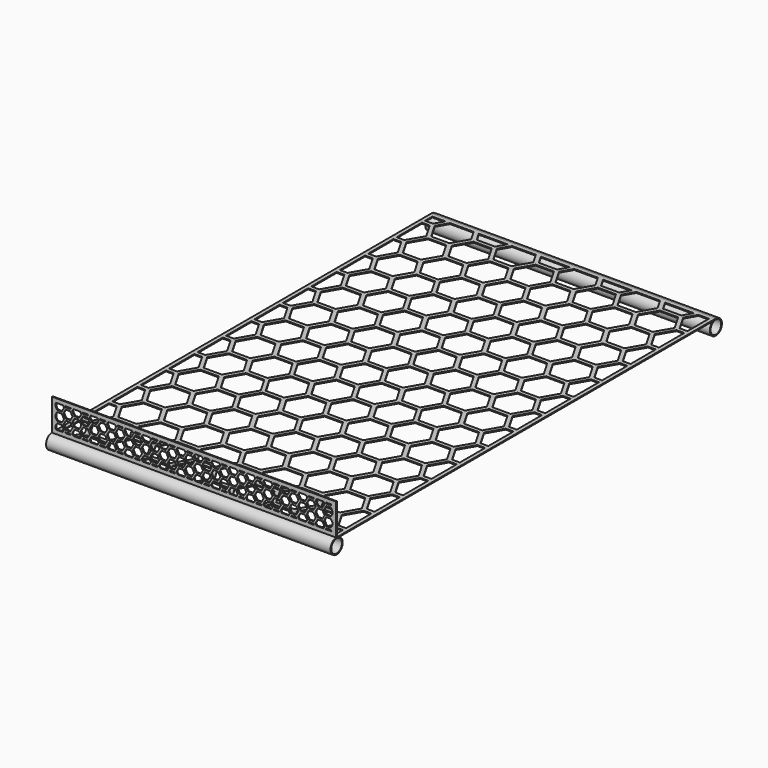
from build123d import *

# Parameters (mm, degrees)
F0_W     = 180
F0_H     = 300
F1_DEPTH = 0.3
F2_R     = 4.2
F2_R_2   = 4.8
F5_DEPTH = 0.6
F7_DEPTH = 490


# Not quite as in the source:
# - an extrude ends at something that could not be found from the text; its depth is read off the source's solid


with BuildPart() as f1:
    # F0 (on Top) → F1 (new body, symmetric)
    with BuildSketch(Plane.XY):
        Rectangle(F0_W, F0_H)
    extrude(amount=F1_DEPTH, both=True)

    # F3: sweep along a path in F3_path
    with BuildLine(Plane(origin=(-90, -150, 0.3), x_dir=(0, 1, 0), z_dir=(0, 0, 1))) as f3_path:
        Line((0, 0), (0, -180))
    # F2 (on Right) → F3 (sweep)
    with BuildSketch(Plane.YZ):
        with BuildLine():
            ThreePointArc((-150.3, 0.2906158268), (-153.286335345, -7.9985711369), (-145.2, -4.5))
            ThreePointArc((-145.2, -4.5), (-146.5014288631, -1.213664655), (-149.7, 0.2906158268))
            Line((-149.7, 0.2906158268), (-150.3, 0.2906158268))
        make_face()
        with Locations((-150, -4.5)):
            Circle(F2_R, mode=Mode.SUBTRACT)
        with BuildLine():
            Line((-150.3, 0.2906158268), (-149.7, 0.2906158268))
            ThreePointArc((-149.7, 0.2906158268), (-150, 0.3), (-150.3, 0.2906158268))
        make_face()
        with BuildLine():
            ThreePointArc((-150.3, 0.2906158268), (-150, 0.3), (-149.7, 0.2906158268))
            Line((-149.7, 0.2906158268), (-149.7, 20.2906158268))
            Line((-149.7, 20.2906158268), (-150.3, 20.2906158268))
            Line((-150.3, 20.2906158268), (-150.3, 0.2906158268))
        make_face()
        with Locations((150, -4.5)):
            Circle(F2_R_2)
        with Locations((150, -4.5)):
            Circle(F2_R, mode=Mode.SUBTRACT)
    sweep(path=f3_path.line)

    # F4 (on face) → F5 (cut, through all)
    with BuildSketch(Plane.XY.offset(0.3)):
        Polygon((-79.2319517736, 147.6762099923), (-87.5, 147.6762099923), (-87.5, 141.875), (-82.5812819243, 141.875), align=None)
        Polygon((-61.3932256344, 147.6762099923), (-76.3452004277, 147.6762099923), (-80.4162184149, 140.625), (-74.642715723, 130.625), (-63.0957103392, 130.625), (-57.3222076473, 140.625), align=None)
        Polygon((-39.9259517736, 147.6762099923), (-58.1716174588, 147.6762099923), (-54.8222873081, 141.875), (-43.2752819243, 141.875), align=None)
        Polygon((-22.0872256344, 147.6762099923), (-37.0392004277, 147.6762099923), (-41.1102184149, 140.625), (-35.336715723, 130.625), (-23.7897103392, 130.625), (-18.0162076473, 140.625), align=None)
        Polygon((-0.6199517736, 147.6762099923), (-18.8656174588, 147.6762099923), (-15.5162873081, 141.875), (-3.9692819243, 141.875), align=None)
        Polygon((17.2187743656, 147.6762099923), (2.2667995723, 147.6762099923), (-1.8042184149, 140.625), (3.969284277, 130.625), (15.5162896608, 130.625), (21.2897923527, 140.625), align=None)
        Polygon((38.6860482264, 147.6762099923), (20.4403825412, 147.6762099923), (23.7897126919, 141.875), (35.3367180757, 141.875), align=None)
        Polygon((56.5247743656, 147.6762099923), (41.5727995723, 147.6762099923), (37.5017815851, 140.625), (43.275284277, 130.625), (54.8222896608, 130.625), (60.5957923527, 140.625), align=None)
        Polygon((77.9920482264, 147.6762099923), (59.7463825412, 147.6762099923), (63.0957126919, 141.875), (74.6427180757, 141.875), align=None)
        Polygon((87.5, 147.6762099923), (80.8787995723, 147.6762099923), (76.8077815851, 140.625), (82.581284277, 130.625), (87.5, 130.625), align=None)
        Polygon((-82.5812819243, 139.375), (-87.5, 139.375), (-87.5, 119.375), (-82.5812819243, 119.375), (-76.8077792324, 129.375), align=None)
        Polygon((-43.2752819243, 139.375), (-54.8222873081, 139.375), (-60.59579, 129.375), (-54.8222873081, 119.375), (-43.2752819243, 119.375), (-37.5017792324, 129.375), align=None)
        Polygon((-3.9692819243, 139.375), (-15.5162873081, 139.375), (-21.28979, 129.375), (-15.5162873081, 119.375), (-3.9692819243, 119.375), (1.8042207676, 129.375), align=None)
        Polygon((35.3367180757, 139.375), (23.7897126919, 139.375), (18.01621, 129.375), (23.7897126919, 119.375), (35.3367180757, 119.375), (41.1102207676, 129.375), align=None)
        Polygon((74.6427180757, 139.375), (63.0957126919, 139.375), (57.32221, 129.375), (63.0957126919, 119.375), (74.6427180757, 119.375), (80.4162207676, 129.375), align=None)
        Polygon((-74.642715723, 128.125), (-80.4162184149, 118.125), (-74.642715723, 108.125), (-63.0957103392, 108.125), (-57.3222076473, 118.125), (-63.0957103392, 128.125), align=None)
        Polygon((-35.336715723, 128.125), (-41.1102184149, 118.125), (-35.336715723, 108.125), (-23.7897103392, 108.125), (-18.0162076473, 118.125), (-23.7897103392, 128.125), align=None)
        Polygon((3.969284277, 128.125), (-1.8042184149, 118.125), (3.969284277, 108.125), (15.5162896608, 108.125), (21.2897923527, 118.125), (15.5162896608, 128.125), align=None)
        Polygon((43.275284277, 128.125), (37.5017815851, 118.125), (43.275284277, 108.125), (54.8222896608, 108.125), (60.5957923527, 118.125), (54.8222896608, 128.125), align=None)
        Polygon((87.5, 108.125), (87.5, 128.125), (82.581284277, 128.125), (76.8077815851, 118.125), (82.581284277, 108.125), align=None)
        Polygon((-82.5812819243, 116.875), (-87.5, 116.875), (-87.5, 96.875), (-82.5812819243, 96.875), (-76.8077792324, 106.875), align=None)
        Polygon((-43.2752819243, 116.875), (-54.8222873081, 116.875), (-60.59579, 106.875), (-54.8222873081, 96.875), (-43.2752819243, 96.875), (-37.5017792324, 106.875), align=None)
        Polygon((-3.9692819243, 116.875), (-15.5162873081, 116.875), (-21.28979, 106.875), (-15.5162873081, 96.875), (-3.9692819243, 96.875), (1.8042207676, 106.875), align=None)
        Polygon((35.3367180757, 116.875), (23.7897126919, 116.875), (18.01621, 106.875), (23.7897126919, 96.875), (35.3367180757, 96.875), (41.1102207676, 106.875), align=None)
        Polygon((74.6427180757, 116.875), (63.0957126919, 116.875), (57.32221, 106.875), (63.0957126919, 96.875), (74.6427180757, 96.875), (80.4162207676, 106.875), align=None)
        Polygon((-74.642715723, 105.625), (-80.4162184149, 95.625), (-74.642715723, 85.625), (-63.0957103392, 85.625), (-57.3222076473, 95.625), (-63.0957103392, 105.625), align=None)
        Polygon((-35.336715723, 105.625), (-41.1102184149, 95.625), (-35.336715723, 85.625), (-23.7897103392, 85.625), (-18.0162076473, 95.625), (-23.7897103392, 105.625), align=None)
        Polygon((3.969284277, 105.625), (-1.8042184149, 95.625), (3.969284277, 85.625), (15.5162896608, 85.625), (21.2897923527, 95.625), (15.5162896608, 105.625), align=None)
        Polygon((43.275284277, 105.625), (37.5017815851, 95.625), (43.275284277, 85.625), (54.8222896608, 85.625), (60.5957923527, 95.625), (54.8222896608, 105.625), align=None)
        Polygon((87.5, 85.625), (87.5, 105.625), (82.581284277, 105.625), (76.8077815851, 95.625), (82.581284277, 85.625), align=None)
        Polygon((-82.5812819243, 94.375), (-87.5, 94.375), (-87.5, 74.375), (-82.5812819243, 74.375), (-76.8077792324, 84.375), align=None)
        Polygon((-43.2752819243, 94.375), (-54.8222873081, 94.375), (-60.59579, 84.375), (-54.8222873081, 74.375), (-43.2752819243, 74.375), (-37.5017792324, 84.375), align=None)
        Polygon((-3.9692819243, 94.375), (-15.5162873081, 94.375), (-21.28979, 84.375), (-15.5162873081, 74.375), (-3.9692819243, 74.375), (1.8042207676, 84.375), align=None)
        Polygon((35.3367180757, 94.375), (23.7897126919, 94.375), (18.01621, 84.375), (23.7897126919, 74.375), (35.3367180757, 74.375), (41.1102207676, 84.375), align=None)
        Polygon((74.6427180757, 94.375), (63.0957126919, 94.375), (57.32221, 84.375), (63.0957126919, 74.375), (74.6427180757, 74.375), (80.4162207676, 84.375), align=None)
        Polygon((-74.642715723, 83.125), (-80.4162184149, 73.125), (-74.642715723, 63.125), (-63.0957103392, 63.125), (-57.3222076473, 73.125), (-63.0957103392, 83.125), align=None)
        Polygon((-35.336715723, 83.125), (-41.1102184149, 73.125), (-35.336715723, 63.125), (-23.7897103392, 63.125), (-18.0162076473, 73.125), (-23.7897103392, 83.125), align=None)
        Polygon((3.969284277, 83.125), (-1.8042184149, 73.125), (3.969284277, 63.125), (15.5162896608, 63.125), (21.2897923527, 73.125), (15.5162896608, 83.125), align=None)
        Polygon((43.275284277, 83.125), (37.5017815851, 73.125), (43.275284277, 63.125), (54.8222896608, 63.125), (60.5957923527, 73.125), (54.8222896608, 83.125), align=None)
        Polygon((87.5, 63.125), (87.5, 83.125), (82.581284277, 83.125), (76.8077815851, 73.125), (82.581284277, 63.125), align=None)
        Polygon((-82.5812819243, 71.875), (-87.5, 71.875), (-87.5, 51.875), (-82.5812819243, 51.875), (-76.8077792324, 61.875), align=None)
        Polygon((-43.2752819243, 71.875), (-54.8222873081, 71.875), (-60.59579, 61.875), (-54.8222873081, 51.875), (-43.2752819243, 51.875), (-37.5017792324, 61.875), align=None)
        Polygon((-3.9692819243, 71.875), (-15.5162873081, 71.875), (-21.28979, 61.875), (-15.5162873081, 51.875), (-3.9692819243, 51.875), (1.8042207676, 61.875), align=None)
        Polygon((35.3367180757, 71.875), (23.7897126919, 71.875), (18.01621, 61.875), (23.7897126919, 51.875), (35.3367180757, 51.875), (41.1102207676, 61.875), align=None)
        Polygon((74.6427180757, 71.875), (63.0957126919, 71.875), (57.32221, 61.875), (63.0957126919, 51.875), (74.6427180757, 51.875), (80.4162207676, 61.875), align=None)
        Polygon((-74.642715723, 60.625), (-80.4162184149, 50.625), (-74.642715723, 40.625), (-63.0957103392, 40.625), (-57.3222076473, 50.625), (-63.0957103392, 60.625), align=None)
        Polygon((-35.336715723, 60.625), (-41.1102184149, 50.625), (-35.336715723, 40.625), (-23.7897103392, 40.625), (-18.0162076473, 50.625), (-23.7897103392, 60.625), align=None)
        Polygon((3.969284277, 60.625), (-1.8042184149, 50.625), (3.969284277, 40.625), (15.5162896608, 40.625), (21.2897923527, 50.625), (15.5162896608, 60.625), align=None)
        Polygon((43.275284277, 60.625), (37.5017815851, 50.625), (43.275284277, 40.625), (54.8222896608, 40.625), (60.5957923527, 50.625), (54.8222896608, 60.625), align=None)
        Polygon((87.5, 40.625), (87.5, 60.625), (82.581284277, 60.625), (76.8077815851, 50.625), (82.581284277, 40.625), align=None)
        Polygon((-82.5812819243, 49.375), (-87.5, 49.375), (-87.5, 29.375), (-82.5812819243, 29.375), (-76.8077792324, 39.375), align=None)
        Polygon((-43.2752819243, 49.375), (-54.8222873081, 49.375), (-60.59579, 39.375), (-54.8222873081, 29.375), (-43.2752819243, 29.375), (-37.5017792324, 39.375), align=None)
        Polygon((-3.9692819243, 49.375), (-15.5162873081, 49.375), (-21.28979, 39.375), (-15.5162873081, 29.375), (-3.9692819243, 29.375), (1.8042207676, 39.375), align=None)
        Polygon((35.3367180757, 49.375), (23.7897126919, 49.375), (18.01621, 39.375), (23.7897126919, 29.375), (35.3367180757, 29.375), (41.1102207676, 39.375), align=None)
        Polygon((74.6427180757, 49.375), (63.0957126919, 49.375), (57.32221, 39.375), (63.0957126919, 29.375), (74.6427180757, 29.375), (80.4162207676, 39.375), align=None)
        Polygon((-74.642715723, 38.125), (-80.4162184149, 28.125), (-74.642715723, 18.125), (-63.0957103392, 18.125), (-57.3222076473, 28.125), (-63.0957103392, 38.125), align=None)
        Polygon((-35.336715723, 38.125), (-41.1102184149, 28.125), (-35.336715723, 18.125), (-23.7897103392, 18.125), (-18.0162076473, 28.125), (-23.7897103392, 38.125), align=None)
        Polygon((3.969284277, 38.125), (-1.8042184149, 28.125), (3.969284277, 18.125), (15.5162896608, 18.125), (21.2897923527, 28.125), (15.5162896608, 38.125), align=None)
        Polygon((43.275284277, 38.125), (37.5017815851, 28.125), (43.275284277, 18.125), (54.8222896608, 18.125), (60.5957923527, 28.125), (54.8222896608, 38.125), align=None)
        Polygon((87.5, 18.125), (87.5, 38.125), (82.581284277, 38.125), (76.8077815851, 28.125), (82.581284277, 18.125), align=None)
        Polygon((-82.5812819243, 26.875), (-87.5, 26.875), (-87.5, 6.875), (-82.5812819243, 6.875), (-76.8077792324, 16.875), align=None)
        Polygon((-43.2752819243, 26.875), (-54.8222873081, 26.875), (-60.59579, 16.875), (-54.8222873081, 6.875), (-43.2752819243, 6.875), (-37.5017792324, 16.875), align=None)
        Polygon((-3.9692819243, 26.875), (-15.5162873081, 26.875), (-21.28979, 16.875), (-15.5162873081, 6.875), (-3.9692819243, 6.875), (1.8042207676, 16.875), align=None)
        Polygon((35.3367180757, 26.875), (23.7897126919, 26.875), (18.01621, 16.875), (23.7897126919, 6.875), (35.3367180757, 6.875), (41.1102207676, 16.875), align=None)
        Polygon((74.6427180757, 26.875), (63.0957126919, 26.875), (57.32221, 16.875), (63.0957126919, 6.875), (74.6427180757, 6.875), (80.4162207676, 16.875), align=None)
        Polygon((-74.642715723, 15.625), (-80.4162184149, 5.625), (-74.642715723, -4.375), (-63.0957103392, -4.375), (-57.3222076473, 5.625), (-63.0957103392, 15.625), align=None)
        Polygon((-35.336715723, 15.625), (-41.1102184149, 5.625), (-35.336715723, -4.375), (-23.7897103392, -4.375), (-18.0162076473, 5.625), (-23.7897103392, 15.625), align=None)
        Polygon((3.969284277, 15.625), (-1.8042184149, 5.625), (3.969284277, -4.375), (15.5162896608, -4.375), (21.2897923527, 5.625), (15.5162896608, 15.625), align=None)
        Polygon((43.275284277, 15.625), (37.5017815851, 5.625), (43.275284277, -4.375), (54.8222896608, -4.375), (60.5957923527, 5.625), (54.8222896608, 15.625), align=None)
        Polygon((87.5, -4.375), (87.5, 15.625), (82.581284277, 15.625), (76.8077815851, 5.625), (82.581284277, -4.375), align=None)
        Polygon((-82.5812819243, 4.375), (-87.5, 4.375), (-87.5, -15.625), (-82.5812819243, -15.625), (-76.8077792324, -5.625), align=None)
        Polygon((-43.2752819243, 4.375), (-54.8222873081, 4.375), (-60.59579, -5.625), (-54.8222873081, -15.625), (-43.2752819243, -15.625), (-37.5017792324, -5.625), align=None)
        Polygon((-3.9692819243, 4.375), (-15.5162873081, 4.375), (-21.28979, -5.625), (-15.5162873081, -15.625), (-3.9692819243, -15.625), (1.8042207676, -5.625), align=None)
        Polygon((35.3367180757, 4.375), (23.7897126919, 4.375), (18.01621, -5.625), (23.7897126919, -15.625), (35.3367180757, -15.625), (41.1102207676, -5.625), align=None)
        Polygon((74.6427180757, 4.375), (63.0957126919, 4.375), (57.32221, -5.625), (63.0957126919, -15.625), (74.6427180757, -15.625), (80.4162207676, -5.625), align=None)
        Polygon((-74.642715723, -6.875), (-80.4162184149, -16.875), (-74.642715723, -26.875), (-63.0957103392, -26.875), (-57.3222076473, -16.875), (-63.0957103392, -6.875), align=None)
        Polygon((-35.336715723, -6.875), (-41.1102184149, -16.875), (-35.336715723, -26.875), (-23.7897103392, -26.875), (-18.0162076473, -16.875), (-23.7897103392, -6.875), align=None)
        Polygon((3.969284277, -6.875), (-1.8042184149, -16.875), (3.969284277, -26.875), (15.5162896608, -26.875), (21.2897923527, -16.875), (15.5162896608, -6.875), align=None)
        Polygon((43.275284277, -6.875), (37.5017815851, -16.875), (43.275284277, -26.875), (54.8222896608, -26.875), (60.5957923527, -16.875), (54.8222896608, -6.875), align=None)
        Polygon((87.5, -26.875), (87.5, -6.875), (82.581284277, -6.875), (76.8077815851, -16.875), (82.581284277, -26.875), align=None)
        Polygon((-82.5812819243, -18.125), (-87.5, -18.125), (-87.5, -38.125), (-82.5812819243, -38.125), (-76.8077792324, -28.125), align=None)
        Polygon((-43.2752819243, -18.125), (-54.8222873081, -18.125), (-60.59579, -28.125), (-54.8222873081, -38.125), (-43.2752819243, -38.125), (-37.5017792324, -28.125), align=None)
        Polygon((-3.9692819243, -18.125), (-15.5162873081, -18.125), (-21.28979, -28.125), (-15.5162873081, -38.125), (-3.9692819243, -38.125), (1.8042207676, -28.125), align=None)
        Polygon((35.3367180757, -18.125), (23.7897126919, -18.125), (18.01621, -28.125), (23.7897126919, -38.125), (35.3367180757, -38.125), (41.1102207676, -28.125), align=None)
        Polygon((74.6427180757, -18.125), (63.0957126919, -18.125), (57.32221, -28.125), (63.0957126919, -38.125), (74.6427180757, -38.125), (80.4162207676, -28.125), align=None)
        Polygon((-74.642715723, -29.375), (-80.4162184149, -39.375), (-74.642715723, -49.375), (-63.0957103392, -49.375), (-57.3222076473, -39.375), (-63.0957103392, -29.375), align=None)
        Polygon((-35.336715723, -29.375), (-41.1102184149, -39.375), (-35.336715723, -49.375), (-23.7897103392, -49.375), (-18.0162076473, -39.375), (-23.7897103392, -29.375), align=None)
        Polygon((3.969284277, -29.375), (-1.8042184149, -39.375), (3.969284277, -49.375), (15.5162896608, -49.375), (21.2897923527, -39.375), (15.5162896608, -29.375), align=None)
        Polygon((43.275284277, -29.375), (37.5017815851, -39.375), (43.275284277, -49.375), (54.8222896608, -49.375), (60.5957923527, -39.375), (54.8222896608, -29.375), align=None)
        Polygon((87.5, -49.375), (87.5, -29.375), (82.581284277, -29.375), (76.8077815851, -39.375), (82.581284277, -49.375), align=None)
        Polygon((-82.5812819243, -40.625), (-87.5, -40.625), (-87.5, -60.625), (-82.5812819243, -60.625), (-76.8077792324, -50.625), align=None)
        Polygon((-43.2752819243, -40.625), (-54.8222873081, -40.625), (-60.59579, -50.625), (-54.8222873081, -60.625), (-43.2752819243, -60.625), (-37.5017792324, -50.625), align=None)
        Polygon((-3.9692819243, -40.625), (-15.5162873081, -40.625), (-21.28979, -50.625), (-15.5162873081, -60.625), (-3.9692819243, -60.625), (1.8042207676, -50.625), align=None)
        Polygon((35.3367180757, -40.625), (23.7897126919, -40.625), (18.01621, -50.625), (23.7897126919, -60.625), (35.3367180757, -60.625), (41.1102207676, -50.625), align=None)
        Polygon((74.6427180757, -40.625), (63.0957126919, -40.625), (57.32221, -50.625), (63.0957126919, -60.625), (74.6427180757, -60.625), (80.4162207676, -50.625), align=None)
        Polygon((-74.642715723, -51.875), (-80.4162184149, -61.875), (-74.642715723, -71.875), (-63.0957103392, -71.875), (-57.3222076473, -61.875), (-63.0957103392, -51.875), align=None)
        Polygon((-35.336715723, -51.875), (-41.1102184149, -61.875), (-35.336715723, -71.875), (-23.7897103392, -71.875), (-18.0162076473, -61.875), (-23.7897103392, -51.875), align=None)
        Polygon((3.969284277, -51.875), (-1.8042184149, -61.875), (3.969284277, -71.875), (15.5162896608, -71.875), (21.2897923527, -61.875), (15.5162896608, -51.875), align=None)
        Polygon((43.275284277, -51.875), (37.5017815851, -61.875), (43.275284277, -71.875), (54.8222896608, -71.875), (60.5957923527, -61.875), (54.8222896608, -51.875), align=None)
        Polygon((87.5, -71.875), (87.5, -51.875), (82.581284277, -51.875), (76.8077815851, -61.875), (82.581284277, -71.875), align=None)
        Polygon((-82.5812819243, -63.125), (-87.5, -63.125), (-87.5, -83.125), (-82.5812819243, -83.125), (-76.8077792324, -73.125), align=None)
        Polygon((-43.2752819243, -63.125), (-54.8222873081, -63.125), (-60.59579, -73.125), (-54.8222873081, -83.125), (-43.2752819243, -83.125), (-37.5017792324, -73.125), align=None)
        Polygon((-3.9692819243, -63.125), (-15.5162873081, -63.125), (-21.28979, -73.125), (-15.5162873081, -83.125), (-3.9692819243, -83.125), (1.8042207676, -73.125), align=None)
        Polygon((35.3367180757, -63.125), (23.7897126919, -63.125), (18.01621, -73.125), (23.7897126919, -83.125), (35.3367180757, -83.125), (41.1102207676, -73.125), align=None)
        Polygon((74.6427180757, -63.125), (63.0957126919, -63.125), (57.32221, -73.125), (63.0957126919, -83.125), (74.6427180757, -83.125), (80.4162207676, -73.125), align=None)
        Polygon((-74.642715723, -74.375), (-80.4162184149, -84.375), (-74.642715723, -94.375), (-63.0957103392, -94.375), (-57.3222076473, -84.375), (-63.0957103392, -74.375), align=None)
        Polygon((-35.336715723, -74.375), (-41.1102184149, -84.375), (-35.336715723, -94.375), (-23.7897103392, -94.375), (-18.0162076473, -84.375), (-23.7897103392, -74.375), align=None)
        Polygon((3.969284277, -74.375), (-1.8042184149, -84.375), (3.969284277, -94.375), (15.5162896608, -94.375), (21.2897923527, -84.375), (15.5162896608, -74.375), align=None)
        Polygon((43.275284277, -74.375), (37.5017815851, -84.375), (43.275284277, -94.375), (54.8222896608, -94.375), (60.5957923527, -84.375), (54.8222896608, -74.375), align=None)
        Polygon((87.5, -94.375), (87.5, -74.375), (82.581284277, -74.375), (76.8077815851, -84.375), (82.581284277, -94.375), align=None)
        Polygon((-82.5812819243, -85.625), (-87.5, -85.625), (-87.5, -105.625), (-82.5812819243, -105.625), (-76.8077792324, -95.625), align=None)
        Polygon((-43.2752819243, -85.625), (-54.8222873081, -85.625), (-60.59579, -95.625), (-54.8222873081, -105.625), (-43.2752819243, -105.625), (-37.5017792324, -95.625), align=None)
        Polygon((-3.9692819243, -85.625), (-15.5162873081, -85.625), (-21.28979, -95.625), (-15.5162873081, -105.625), (-3.9692819243, -105.625), (1.8042207676, -95.625), align=None)
        Polygon((35.3367180757, -85.625), (23.7897126919, -85.625), (18.01621, -95.625), (23.7897126919, -105.625), (35.3367180757, -105.625), (41.1102207676, -95.625), align=None)
        Polygon((74.6427180757, -85.625), (63.0957126919, -85.625), (57.32221, -95.625), (63.0957126919, -105.625), (74.6427180757, -105.625), (80.4162207676, -95.625), align=None)
        Polygon((-74.642715723, -96.875), (-80.4162184149, -106.875), (-74.642715723, -116.875), (-63.0957103392, -116.875), (-57.3222076473, -106.875), (-63.0957103392, -96.875), align=None)
        Polygon((-35.336715723, -96.875), (-41.1102184149, -106.875), (-35.336715723, -116.875), (-23.7897103392, -116.875), (-18.0162076473, -106.875), (-23.7897103392, -96.875), align=None)
        Polygon((3.969284277, -96.875), (-1.8042184149, -106.875), (3.969284277, -116.875), (15.5162896608, -116.875), (21.2897923527, -106.875), (15.5162896608, -96.875), align=None)
        Polygon((43.275284277, -96.875), (37.5017815851, -106.875), (43.275284277, -116.875), (54.8222896608, -116.875), (60.5957923527, -106.875), (54.8222896608, -96.875), align=None)
        Polygon((87.5, -116.875), (87.5, -96.875), (82.581284277, -96.875), (76.8077815851, -106.875), (82.581284277, -116.875), align=None)
        Polygon((-82.5812819243, -108.125), (-87.5, -108.125), (-87.5, -128.125), (-82.5812819243, -128.125), (-76.8077792324, -118.125), align=None)
        Polygon((-43.2752819243, -108.125), (-54.8222873081, -108.125), (-60.59579, -118.125), (-54.8222873081, -128.125), (-43.2752819243, -128.125), (-37.5017792324, -118.125), align=None)
        Polygon((-3.9692819243, -108.125), (-15.5162873081, -108.125), (-21.28979, -118.125), (-15.5162873081, -128.125), (-3.9692819243, -128.125), (1.8042207676, -118.125), align=None)
        Polygon((35.3367180757, -108.125), (23.7897126919, -108.125), (18.01621, -118.125), (23.7897126919, -128.125), (35.3367180757, -128.125), (41.1102207676, -118.125), align=None)
        Polygon((74.6427180757, -108.125), (63.0957126919, -108.125), (57.32221, -118.125), (63.0957126919, -128.125), (74.6427180757, -128.125), (80.4162207676, -118.125), align=None)
        Polygon((-74.642715723, -119.375), (-80.4162184149, -129.375), (-74.642715723, -139.375), (-63.0957103392, -139.375), (-57.3222076473, -129.375), (-63.0957103392, -119.375), align=None)
        Polygon((-35.336715723, -119.375), (-41.1102184149, -129.375), (-35.336715723, -139.375), (-23.7897103392, -139.375), (-18.0162076473, -129.375), (-23.7897103392, -119.375), align=None)
        Polygon((3.969284277, -119.375), (-1.8042184149, -129.375), (3.969284277, -139.375), (15.5162896608, -139.375), (21.2897923527, -129.375), (15.5162896608, -119.375), align=None)
        Polygon((43.275284277, -119.375), (37.5017815851, -129.375), (43.275284277, -139.375), (54.8222896608, -139.375), (60.5957923527, -129.375), (54.8222896608, -119.375), align=None)
        Polygon((87.5, -139.375), (87.5, -119.375), (82.581284277, -119.375), (76.8077815851, -129.375), (82.581284277, -139.375), align=None)
        Polygon((-82.5812819243, -130.625), (-87.5, -130.625), (-87.5, -147.6762099923), (-80.8787972196, -147.6762099923), (-76.8077792324, -140.625), align=None)
        Polygon((-74.642715723, -141.875), (-77.9920458736, -147.6762099923), (-59.7463801885, -147.6762099923), (-63.0957103392, -141.875), align=None)
        Polygon((-35.336715723, -141.875), (-38.6860458736, -147.6762099923), (-20.4403801885, -147.6762099923), (-23.7897103392, -141.875), align=None)
        Polygon((-21.28979, -140.625), (-17.2187720128, -147.6762099923), (-2.2667972196, -147.6762099923), (1.8042207676, -140.625), (-3.9692819243, -130.625), (-15.5162873081, -130.625), align=None)
        Polygon((3.969284277, -141.875), (0.6199541264, -147.6762099923), (18.8656198115, -147.6762099923), (15.5162896608, -141.875), align=None)
        Polygon((18.01621, -140.625), (22.0872279872, -147.6762099923), (37.0392027804, -147.6762099923), (41.1102207676, -140.625), (35.3367180757, -130.625), (23.7897126919, -130.625), align=None)
        Polygon((43.275284277, -141.875), (39.9259541264, -147.6762099923), (58.1716198115, -147.6762099923), (54.8222896608, -141.875), align=None)
        Polygon((57.32221, -140.625), (61.3932279872, -147.6762099923), (76.3452027804, -147.6762099923), (80.4162207676, -140.625), (74.6427180757, -130.625), (63.0957126919, -130.625), align=None)
        Polygon((87.5, -147.6762099923), (87.5, -141.875), (82.581284277, -141.875), (79.2319541264, -147.6762099923), align=None)
        Polygon((-60.59579, -140.625), (-56.5247720128, -147.6762099923), (-41.5727972196, -147.6762099923), (-37.5017792324, -140.625), (-43.2752819243, -130.625), (-54.8222873081, -130.625), align=None)
    extrude(amount=-F5_DEPTH, mode=Mode.SUBTRACT)

    # F6 (on face) → F7 (cut, through all)
    with BuildSketch(Plane.XZ.offset(150.3)):
        Polygon((-82.9886851446, 17.7906158268), (-87.3188121635, 17.7906158268), (-87.5, 17.4767892883), (-87.5, 15.6044423653), (-86.597124327, 14.0406158268), (-83.7103729811, 14.0406158268), (-82.2669973081, 16.5406158268), align=None)
        Polygon((-86.597124327, 12.7906158268), (-87.5, 11.2267892883), (-87.5, 9.3544423653), (-86.597124327, 7.7906158268), (-83.7103729811, 7.7906158268), (-82.2669973081, 10.2906158268), (-83.7103729811, 12.7906158268), align=None)
        Polygon((-86.597124327, 6.5406158268), (-87.5, 4.9767892883), (-87.5, 3.1044423653), (-87.3188121635, 2.7906158268), (-82.9886851446, 2.7906158268), (-82.2669973081, 4.0406158268), (-83.7103729811, 6.5406158268), align=None)
        Polygon((-77.9368702892, 17.7906158268), (-81.5453094716, 17.7906158268), (-81.1844655534, 17.1656158268), (-78.2977142074, 17.1656158268), align=None)
        Polygon((-82.6278412263, 13.4156158268), (-81.1844655534, 10.9156158268), (-78.2977142074, 10.9156158268), (-76.8543385345, 13.4156158268), (-78.2977142074, 15.9156158268), (-81.1844655534, 15.9156158268), align=None)
        Polygon((-82.6278412263, 7.1656158268), (-81.1844655534, 4.6656158268), (-78.2977142074, 4.6656158268), (-76.8543385345, 7.1656158268), (-78.2977142074, 9.6656158268), (-81.1844655534, 9.6656158268), align=None)
        Polygon((-81.1844655534, 3.4156158268), (-81.5453094716, 2.7906158268), (-77.9368702892, 2.7906158268), (-78.2977142074, 3.4156158268), align=None)
        Polygon((-71.9956851446, 17.7906158268), (-76.3258121635, 17.7906158268), (-77.0475, 16.5406158268), (-75.604124327, 14.0406158268), (-72.7173729811, 14.0406158268), (-71.2739973081, 16.5406158268), align=None)
        Polygon((-72.7173729811, 12.7906158268), (-75.604124327, 12.7906158268), (-77.0475, 10.2906158268), (-75.604124327, 7.7906158268), (-72.7173729811, 7.7906158268), (-71.2739973081, 10.2906158268), align=None)
        Polygon((-77.0475, 4.0406158268), (-76.3258121635, 2.7906158268), (-71.9956851446, 2.7906158268), (-71.2739973081, 4.0406158268), (-72.7173729811, 6.5406158268), (-75.604124327, 6.5406158268), align=None)
        Polygon((-66.9438702892, 17.7906158268), (-70.5523094716, 17.7906158268), (-70.1914655534, 17.1656158268), (-67.3047142074, 17.1656158268), align=None)
        Polygon((-71.6348412263, 13.4156158268), (-70.1914655534, 10.9156158268), (-67.3047142074, 10.9156158268), (-65.8613385345, 13.4156158268), (-67.3047142074, 15.9156158268), (-70.1914655534, 15.9156158268), align=None)
        Polygon((-71.6348412263, 7.1656158268), (-70.1914655534, 4.6656158268), (-67.3047142074, 4.6656158268), (-65.8613385345, 7.1656158268), (-67.3047142074, 9.6656158268), (-70.1914655534, 9.6656158268), align=None)
        Polygon((-70.1914655534, 3.4156158268), (-70.5523094716, 2.7906158268), (-66.9438702892, 2.7906158268), (-67.3047142074, 3.4156158268), align=None)
        Polygon((-61.0026851446, 17.7906158268), (-65.3328121635, 17.7906158268), (-66.0545, 16.5406158268), (-64.611124327, 14.0406158268), (-61.7243729811, 14.0406158268), (-60.2809973081, 16.5406158268), align=None)
        Polygon((-61.7243729811, 12.7906158268), (-64.611124327, 12.7906158268), (-66.0545, 10.2906158268), (-64.611124327, 7.7906158268), (-61.7243729811, 7.7906158268), (-60.2809973081, 10.2906158268), align=None)
        Polygon((-66.0545, 4.0406158268), (-65.3328121635, 2.7906158268), (-61.0026851446, 2.7906158268), (-60.2809973081, 4.0406158268), (-61.7243729811, 6.5406158268), (-64.611124327, 6.5406158268), align=None)
        Polygon((-55.9508702892, 17.7906158268), (-59.5593094716, 17.7906158268), (-59.1984655534, 17.1656158268), (-56.3117142074, 17.1656158268), align=None)
        Polygon((-60.6418412263, 13.4156158268), (-59.1984655534, 10.9156158268), (-56.3117142074, 10.9156158268), (-54.8683385345, 13.4156158268), (-56.3117142074, 15.9156158268), (-59.1984655534, 15.9156158268), align=None)
        Polygon((-60.6418412263, 7.1656158268), (-59.1984655534, 4.6656158268), (-56.3117142074, 4.6656158268), (-54.8683385345, 7.1656158268), (-56.3117142074, 9.6656158268), (-59.1984655534, 9.6656158268), align=None)
        Polygon((-59.1984655534, 3.4156158268), (-59.5593094716, 2.7906158268), (-55.9508702892, 2.7906158268), (-56.3117142074, 3.4156158268), align=None)
        Polygon((-50.0096851446, 17.7906158268), (-54.3398121635, 17.7906158268), (-55.0615, 16.5406158268), (-53.618124327, 14.0406158268), (-50.7313729811, 14.0406158268), (-49.2879973081, 16.5406158268), align=None)
        Polygon((-50.7313729811, 12.7906158268), (-53.618124327, 12.7906158268), (-55.0615, 10.2906158268), (-53.618124327, 7.7906158268), (-50.7313729811, 7.7906158268), (-49.2879973081, 10.2906158268), align=None)
        Polygon((-55.0615, 4.0406158268), (-54.3398121635, 2.7906158268), (-50.0096851446, 2.7906158268), (-49.2879973081, 4.0406158268), (-50.7313729811, 6.5406158268), (-53.618124327, 6.5406158268), align=None)
        Polygon((-44.9578702892, 17.7906158268), (-48.5663094716, 17.7906158268), (-48.2054655534, 17.1656158268), (-45.3187142074, 17.1656158268), align=None)
        Polygon((-49.6488412263, 13.4156158268), (-48.2054655534, 10.9156158268), (-45.3187142074, 10.9156158268), (-43.8753385345, 13.4156158268), (-45.3187142074, 15.9156158268), (-48.2054655534, 15.9156158268), align=None)
        Polygon((-49.6488412263, 7.1656158268), (-48.2054655534, 4.6656158268), (-45.3187142074, 4.6656158268), (-43.8753385345, 7.1656158268), (-45.3187142074, 9.6656158268), (-48.2054655534, 9.6656158268), align=None)
        Polygon((-48.2054655534, 3.4156158268), (-48.5663094716, 2.7906158268), (-44.9578702892, 2.7906158268), (-45.3187142074, 3.4156158268), align=None)
        Polygon((-39.0166851446, 17.7906158268), (-43.3468121635, 17.7906158268), (-44.0685, 16.5406158268), (-42.625124327, 14.0406158268), (-39.7383729811, 14.0406158268), (-38.2949973081, 16.5406158268), align=None)
        Polygon((-39.7383729811, 12.7906158268), (-42.625124327, 12.7906158268), (-44.0685, 10.2906158268), (-42.625124327, 7.7906158268), (-39.7383729811, 7.7906158268), (-38.2949973081, 10.2906158268), align=None)
        Polygon((-44.0685, 4.0406158268), (-43.3468121635, 2.7906158268), (-39.0166851446, 2.7906158268), (-38.2949973081, 4.0406158268), (-39.7383729811, 6.5406158268), (-42.625124327, 6.5406158268), align=None)
        Polygon((-33.9648702892, 17.7906158268), (-37.5733094716, 17.7906158268), (-37.2124655534, 17.1656158268), (-34.3257142074, 17.1656158268), align=None)
        Polygon((-38.6558412263, 13.4156158268), (-37.2124655534, 10.9156158268), (-34.3257142074, 10.9156158268), (-32.8823385345, 13.4156158268), (-34.3257142074, 15.9156158268), (-37.2124655534, 15.9156158268), align=None)
        Polygon((-38.6558412263, 7.1656158268), (-37.2124655534, 4.6656158268), (-34.3257142074, 4.6656158268), (-32.8823385345, 7.1656158268), (-34.3257142074, 9.6656158268), (-37.2124655534, 9.6656158268), align=None)
        Polygon((-37.2124655534, 3.4156158268), (-37.5733094716, 2.7906158268), (-33.9648702892, 2.7906158268), (-34.3257142074, 3.4156158268), align=None)
        Polygon((-28.0236851446, 17.7906158268), (-32.3538121635, 17.7906158268), (-33.0755, 16.5406158268), (-31.632124327, 14.0406158268), (-28.7453729811, 14.0406158268), (-27.3019973081, 16.5406158268), align=None)
        Polygon((-28.7453729811, 12.7906158268), (-31.632124327, 12.7906158268), (-33.0755, 10.2906158268), (-31.632124327, 7.7906158268), (-28.7453729811, 7.7906158268), (-27.3019973081, 10.2906158268), align=None)
        Polygon((-33.0755, 4.0406158268), (-32.3538121635, 2.7906158268), (-28.0236851446, 2.7906158268), (-27.3019973081, 4.0406158268), (-28.7453729811, 6.5406158268), (-31.632124327, 6.5406158268), align=None)
        Polygon((-22.9718702892, 17.7906158268), (-26.5803094716, 17.7906158268), (-26.2194655534, 17.1656158268), (-23.3327142074, 17.1656158268), align=None)
        Polygon((-27.6628412263, 13.4156158268), (-26.2194655534, 10.9156158268), (-23.3327142074, 10.9156158268), (-21.8893385345, 13.4156158268), (-23.3327142074, 15.9156158268), (-26.2194655534, 15.9156158268), align=None)
        Polygon((-27.6628412263, 7.1656158268), (-26.2194655534, 4.6656158268), (-23.3327142074, 4.6656158268), (-21.8893385345, 7.1656158268), (-23.3327142074, 9.6656158268), (-26.2194655534, 9.6656158268), align=None)
        Polygon((-26.2194655534, 3.4156158268), (-26.5803094716, 2.7906158268), (-22.9718702892, 2.7906158268), (-23.3327142074, 3.4156158268), align=None)
        Polygon((-17.0306851446, 17.7906158268), (-21.3608121635, 17.7906158268), (-22.0825, 16.5406158268), (-20.639124327, 14.0406158268), (-17.7523729811, 14.0406158268), (-16.3089973081, 16.5406158268), align=None)
        Polygon((-17.7523729811, 12.7906158268), (-20.639124327, 12.7906158268), (-22.0825, 10.2906158268), (-20.639124327, 7.7906158268), (-17.7523729811, 7.7906158268), (-16.3089973081, 10.2906158268), align=None)
        Polygon((-22.0825, 4.0406158268), (-21.3608121635, 2.7906158268), (-17.0306851446, 2.7906158268), (-16.3089973081, 4.0406158268), (-17.7523729811, 6.5406158268), (-20.639124327, 6.5406158268), align=None)
        Polygon((-11.9788702892, 17.7906158268), (-15.5873094716, 17.7906158268), (-15.2264655534, 17.1656158268), (-12.3397142074, 17.1656158268), align=None)
        Polygon((-16.6698412263, 13.4156158268), (-15.2264655534, 10.9156158268), (-12.3397142074, 10.9156158268), (-10.8963385345, 13.4156158268), (-12.3397142074, 15.9156158268), (-15.2264655534, 15.9156158268), align=None)
        Polygon((-16.6698412263, 7.1656158268), (-15.2264655534, 4.6656158268), (-12.3397142074, 4.6656158268), (-10.8963385345, 7.1656158268), (-12.3397142074, 9.6656158268), (-15.2264655534, 9.6656158268), align=None)
        Polygon((-15.2264655534, 3.4156158268), (-15.5873094716, 2.7906158268), (-11.9788702892, 2.7906158268), (-12.3397142074, 3.4156158268), align=None)
        Polygon((-6.0376851446, 17.7906158268), (-10.3678121635, 17.7906158268), (-11.0895, 16.5406158268), (-9.646124327, 14.0406158268), (-6.7593729811, 14.0406158268), (-5.3159973081, 16.5406158268), align=None)
        Polygon((-6.7593729811, 12.7906158268), (-9.646124327, 12.7906158268), (-11.0895, 10.2906158268), (-9.646124327, 7.7906158268), (-6.7593729811, 7.7906158268), (-5.3159973081, 10.2906158268), align=None)
        Polygon((-11.0895, 4.0406158268), (-10.3678121635, 2.7906158268), (-6.0376851446, 2.7906158268), (-5.3159973081, 4.0406158268), (-6.7593729811, 6.5406158268), (-9.646124327, 6.5406158268), align=None)
        Polygon((-0.9858702892, 17.7906158268), (-4.5943094716, 17.7906158268), (-4.2334655534, 17.1656158268), (-1.3467142074, 17.1656158268), align=None)
        Polygon((-5.6768412263, 13.4156158268), (-4.2334655534, 10.9156158268), (-1.3467142074, 10.9156158268), (0.0966614655, 13.4156158268), (-1.3467142074, 15.9156158268), (-4.2334655534, 15.9156158268), align=None)
        Polygon((-5.6768412263, 7.1656158268), (-4.2334655534, 4.6656158268), (-1.3467142074, 4.6656158268), (0.0966614655, 7.1656158268), (-1.3467142074, 9.6656158268), (-4.2334655534, 9.6656158268), align=None)
        Polygon((-4.2334655534, 3.4156158268), (-4.5943094716, 2.7906158268), (-0.9858702892, 2.7906158268), (-1.3467142074, 3.4156158268), align=None)
        Polygon((4.9553148554, 17.7906158268), (0.6251878365, 17.7906158268), (-0.0965, 16.5406158268), (1.346875673, 14.0406158268), (4.2336270189, 14.0406158268), (5.6770026919, 16.5406158268), align=None)
        Polygon((4.2336270189, 12.7906158268), (1.346875673, 12.7906158268), (-0.0965, 10.2906158268), (1.346875673, 7.7906158268), (4.2336270189, 7.7906158268), (5.6770026919, 10.2906158268), align=None)
        Polygon((-0.0965, 4.0406158268), (0.6251878365, 2.7906158268), (4.9553148554, 2.7906158268), (5.6770026919, 4.0406158268), (4.2336270189, 6.5406158268), (1.346875673, 6.5406158268), align=None)
        Polygon((10.0071297108, 17.7906158268), (6.3986905284, 17.7906158268), (6.7595344466, 17.1656158268), (9.6462857926, 17.1656158268), align=None)
        Polygon((5.3161587737, 13.4156158268), (6.7595344466, 10.9156158268), (9.6462857926, 10.9156158268), (11.0896614655, 13.4156158268), (9.6462857926, 15.9156158268), (6.7595344466, 15.9156158268), align=None)
        Polygon((5.3161587737, 7.1656158268), (6.7595344466, 4.6656158268), (9.6462857926, 4.6656158268), (11.0896614655, 7.1656158268), (9.6462857926, 9.6656158268), (6.7595344466, 9.6656158268), align=None)
        Polygon((6.7595344466, 3.4156158268), (6.3986905284, 2.7906158268), (10.0071297108, 2.7906158268), (9.6462857926, 3.4156158268), align=None)
        Polygon((15.9483148554, 17.7906158268), (11.6181878365, 17.7906158268), (10.8965, 16.5406158268), (12.339875673, 14.0406158268), (15.2266270189, 14.0406158268), (16.6700026919, 16.5406158268), align=None)
        Polygon((15.2266270189, 12.7906158268), (12.339875673, 12.7906158268), (10.8965, 10.2906158268), (12.339875673, 7.7906158268), (15.2266270189, 7.7906158268), (16.6700026919, 10.2906158268), align=None)
        Polygon((10.8965, 4.0406158268), (11.6181878365, 2.7906158268), (15.9483148554, 2.7906158268), (16.6700026919, 4.0406158268), (15.2266270189, 6.5406158268), (12.339875673, 6.5406158268), align=None)
        Polygon((21.0001297108, 17.7906158268), (17.3916905284, 17.7906158268), (17.7525344466, 17.1656158268), (20.6392857926, 17.1656158268), align=None)
        Polygon((16.3091587737, 13.4156158268), (17.7525344466, 10.9156158268), (20.6392857926, 10.9156158268), (22.0826614655, 13.4156158268), (20.6392857926, 15.9156158268), (17.7525344466, 15.9156158268), align=None)
        Polygon((16.3091587737, 7.1656158268), (17.7525344466, 4.6656158268), (20.6392857926, 4.6656158268), (22.0826614655, 7.1656158268), (20.6392857926, 9.6656158268), (17.7525344466, 9.6656158268), align=None)
        Polygon((17.7525344466, 3.4156158268), (17.3916905284, 2.7906158268), (21.0001297108, 2.7906158268), (20.6392857926, 3.4156158268), align=None)
        Polygon((26.9413148554, 17.7906158268), (22.6111878365, 17.7906158268), (21.8895, 16.5406158268), (23.332875673, 14.0406158268), (26.2196270189, 14.0406158268), (27.6630026919, 16.5406158268), align=None)
        Polygon((26.2196270189, 12.7906158268), (23.332875673, 12.7906158268), (21.8895, 10.2906158268), (23.332875673, 7.7906158268), (26.2196270189, 7.7906158268), (27.6630026919, 10.2906158268), align=None)
        Polygon((21.8895, 4.0406158268), (22.6111878365, 2.7906158268), (26.9413148554, 2.7906158268), (27.6630026919, 4.0406158268), (26.2196270189, 6.5406158268), (23.332875673, 6.5406158268), align=None)
        Polygon((31.9931297108, 17.7906158268), (28.3846905284, 17.7906158268), (28.7455344466, 17.1656158268), (31.6322857926, 17.1656158268), align=None)
        Polygon((27.3021587737, 13.4156158268), (28.7455344466, 10.9156158268), (31.6322857926, 10.9156158268), (33.0756614655, 13.4156158268), (31.6322857926, 15.9156158268), (28.7455344466, 15.9156158268), align=None)
        Polygon((27.3021587737, 7.1656158268), (28.7455344466, 4.6656158268), (31.6322857926, 4.6656158268), (33.0756614655, 7.1656158268), (31.6322857926, 9.6656158268), (28.7455344466, 9.6656158268), align=None)
        Polygon((28.7455344466, 3.4156158268), (28.3846905284, 2.7906158268), (31.9931297108, 2.7906158268), (31.6322857926, 3.4156158268), align=None)
        Polygon((37.9343148554, 17.7906158268), (33.6041878365, 17.7906158268), (32.8825, 16.5406158268), (34.325875673, 14.0406158268), (37.2126270189, 14.0406158268), (38.6560026919, 16.5406158268), align=None)
        Polygon((37.2126270189, 12.7906158268), (34.325875673, 12.7906158268), (32.8825, 10.2906158268), (34.325875673, 7.7906158268), (37.2126270189, 7.7906158268), (38.6560026919, 10.2906158268), align=None)
        Polygon((32.8825, 4.0406158268), (33.6041878365, 2.7906158268), (37.9343148554, 2.7906158268), (38.6560026919, 4.0406158268), (37.2126270189, 6.5406158268), (34.325875673, 6.5406158268), align=None)
        Polygon((42.9861297108, 17.7906158268), (39.3776905284, 17.7906158268), (39.7385344466, 17.1656158268), (42.6252857926, 17.1656158268), align=None)
        Polygon((38.2951587737, 13.4156158268), (39.7385344466, 10.9156158268), (42.6252857926, 10.9156158268), (44.0686614655, 13.4156158268), (42.6252857926, 15.9156158268), (39.7385344466, 15.9156158268), align=None)
        Polygon((38.2951587737, 7.1656158268), (39.7385344466, 4.6656158268), (42.6252857926, 4.6656158268), (44.0686614655, 7.1656158268), (42.6252857926, 9.6656158268), (39.7385344466, 9.6656158268), align=None)
        Polygon((39.7385344466, 3.4156158268), (39.3776905284, 2.7906158268), (42.9861297108, 2.7906158268), (42.6252857926, 3.4156158268), align=None)
        Polygon((48.9273148554, 17.7906158268), (44.5971878365, 17.7906158268), (43.8755, 16.5406158268), (45.318875673, 14.0406158268), (48.2056270189, 14.0406158268), (49.6490026919, 16.5406158268), align=None)
        Polygon((48.2056270189, 12.7906158268), (45.318875673, 12.7906158268), (43.8755, 10.2906158268), (45.318875673, 7.7906158268), (48.2056270189, 7.7906158268), (49.6490026919, 10.2906158268), align=None)
        Polygon((43.8755, 4.0406158268), (44.5971878365, 2.7906158268), (48.9273148554, 2.7906158268), (49.6490026919, 4.0406158268), (48.2056270189, 6.5406158268), (45.318875673, 6.5406158268), align=None)
        Polygon((53.9791297108, 17.7906158268), (50.3706905284, 17.7906158268), (50.7315344466, 17.1656158268), (53.6182857926, 17.1656158268), align=None)
        Polygon((49.2881587737, 13.4156158268), (50.7315344466, 10.9156158268), (53.6182857926, 10.9156158268), (55.0616614655, 13.4156158268), (53.6182857926, 15.9156158268), (50.7315344466, 15.9156158268), align=None)
        Polygon((49.2881587737, 7.1656158268), (50.7315344466, 4.6656158268), (53.6182857926, 4.6656158268), (55.0616614655, 7.1656158268), (53.6182857926, 9.6656158268), (50.7315344466, 9.6656158268), align=None)
        Polygon((50.7315344466, 3.4156158268), (50.3706905284, 2.7906158268), (53.9791297108, 2.7906158268), (53.6182857926, 3.4156158268), align=None)
        Polygon((59.9203148554, 17.7906158268), (55.5901878365, 17.7906158268), (54.8685, 16.5406158268), (56.311875673, 14.0406158268), (59.1986270189, 14.0406158268), (60.6420026919, 16.5406158268), align=None)
        Polygon((59.1986270189, 12.7906158268), (56.311875673, 12.7906158268), (54.8685, 10.2906158268), (56.311875673, 7.7906158268), (59.1986270189, 7.7906158268), (60.6420026919, 10.2906158268), align=None)
        Polygon((54.8685, 4.0406158268), (55.5901878365, 2.7906158268), (59.9203148554, 2.7906158268), (60.6420026919, 4.0406158268), (59.1986270189, 6.5406158268), (56.311875673, 6.5406158268), align=None)
        Polygon((64.9721297108, 17.7906158268), (61.3636905284, 17.7906158268), (61.7245344466, 17.1656158268), (64.6112857926, 17.1656158268), align=None)
        Polygon((60.2811587737, 13.4156158268), (61.7245344466, 10.9156158268), (64.6112857926, 10.9156158268), (66.0546614655, 13.4156158268), (64.6112857926, 15.9156158268), (61.7245344466, 15.9156158268), align=None)
        Polygon((60.2811587737, 7.1656158268), (61.7245344466, 4.6656158268), (64.6112857926, 4.6656158268), (66.0546614655, 7.1656158268), (64.6112857926, 9.6656158268), (61.7245344466, 9.6656158268), align=None)
        Polygon((61.7245344466, 3.4156158268), (61.3636905284, 2.7906158268), (64.9721297108, 2.7906158268), (64.6112857926, 3.4156158268), align=None)
        Polygon((70.9133148554, 17.7906158268), (66.5831878365, 17.7906158268), (65.8615, 16.5406158268), (67.304875673, 14.0406158268), (70.1916270189, 14.0406158268), (71.6350026919, 16.5406158268), align=None)
        Polygon((70.1916270189, 12.7906158268), (67.304875673, 12.7906158268), (65.8615, 10.2906158268), (67.304875673, 7.7906158268), (70.1916270189, 7.7906158268), (71.6350026919, 10.2906158268), align=None)
        Polygon((65.8615, 4.0406158268), (66.5831878365, 2.7906158268), (70.9133148554, 2.7906158268), (71.6350026919, 4.0406158268), (70.1916270189, 6.5406158268), (67.304875673, 6.5406158268), align=None)
        Polygon((75.9651297108, 17.7906158268), (72.3566905284, 17.7906158268), (72.7175344466, 17.1656158268), (75.6042857926, 17.1656158268), align=None)
        Polygon((71.2741587737, 13.4156158268), (72.7175344466, 10.9156158268), (75.6042857926, 10.9156158268), (77.0476614655, 13.4156158268), (75.6042857926, 15.9156158268), (72.7175344466, 15.9156158268), align=None)
        Polygon((71.2741587737, 7.1656158268), (72.7175344466, 4.6656158268), (75.6042857926, 4.6656158268), (77.0476614655, 7.1656158268), (75.6042857926, 9.6656158268), (72.7175344466, 9.6656158268), align=None)
        Polygon((72.7175344466, 3.4156158268), (72.3566905284, 2.7906158268), (75.9651297108, 2.7906158268), (75.6042857926, 3.4156158268), align=None)
        Polygon((81.9063148554, 17.7906158268), (77.5761878365, 17.7906158268), (76.8545, 16.5406158268), (78.297875673, 14.0406158268), (81.1846270189, 14.0406158268), (82.6280026919, 16.5406158268), align=None)
        Polygon((81.1846270189, 12.7906158268), (78.297875673, 12.7906158268), (76.8545, 10.2906158268), (78.297875673, 7.7906158268), (81.1846270189, 7.7906158268), (82.6280026919, 10.2906158268), align=None)
        Polygon((76.8545, 4.0406158268), (77.5761878365, 2.7906158268), (81.9063148554, 2.7906158268), (82.6280026919, 4.0406158268), (81.1846270189, 6.5406158268), (78.297875673, 6.5406158268), align=None)
        Polygon((86.9581297108, 17.7906158268), (83.3496905284, 17.7906158268), (83.7105344466, 17.1656158268), (86.5972857926, 17.1656158268), align=None)
        Polygon((87.5, 12.4791626988), (87.5, 14.3520689548), (86.5972857926, 15.9156158268), (83.7105344466, 15.9156158268), (82.2671587737, 13.4156158268), (83.7105344466, 10.9156158268), (86.5972857926, 10.9156158268), align=None)
        Polygon((87.5, 6.2291626988), (87.5, 8.1020689548), (86.5972857926, 9.6656158268), (83.7105344466, 9.6656158268), (82.2671587737, 7.1656158268), (83.7105344466, 4.6656158268), (86.5972857926, 4.6656158268), align=None)
        Polygon((83.7105344466, 3.4156158268), (83.3496905284, 2.7906158268), (86.9581297108, 2.7906158268), (86.5972857926, 3.4156158268), align=None)
    extrude(amount=-F7_DEPTH, mode=Mode.SUBTRACT)


solid = f1.part
